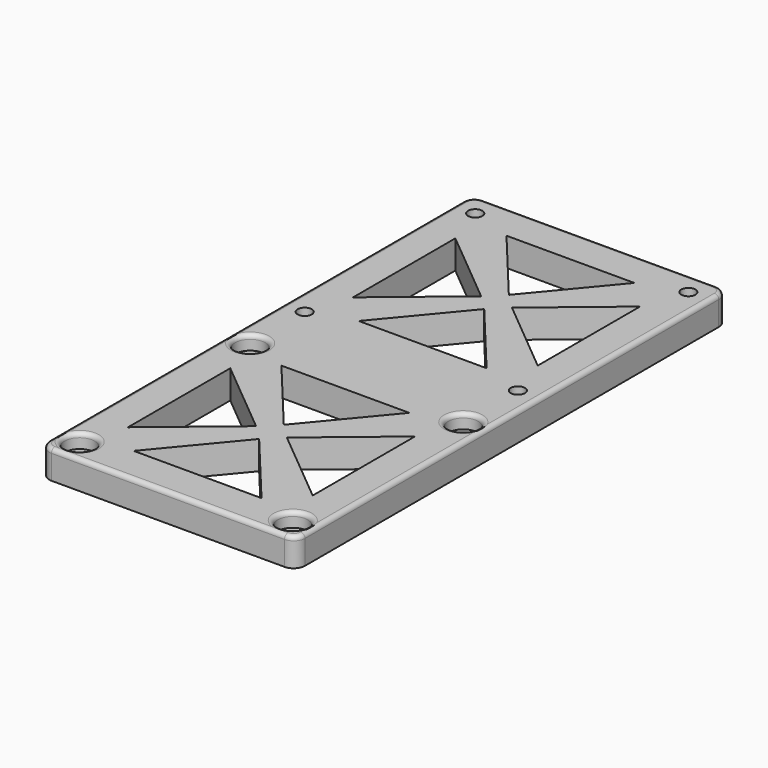
from build123d import *

# Parameters (mm, degrees)
F0_W         = 90
F0_H         = 190
F0_R         = 2.5
F1_DEPTH     = 10
F2_R         = 5.25
F3_DEPTH     = 5
F4_T1_DEPTH  = 197.5
F4_T3_DEPTH  = 97.5
F5_T1_DEPTH  = 19.9999999999
F5_T4_ANGLE  = 90
F5_T6_ANGLE  = 90
F5_T8_ANGLE  = 90
F5_T10_ANGLE = 90
F7_DEPTH     = 10


# Not quite as in the source:
# - a fillet or chamfer that OpenCascade refuses, or shapes differently, is made with other operations: its cross-section is extruded or revolved along the edge and cut away or added


with BuildPart() as f1:
    # F0 (on Top) → F1 (new body)
    with BuildSketch(Plane.XY):
        Rectangle(F0_W, F0_H)
        with Locations((-37.5, -87)):
            Circle(F0_R, mode=Mode.SUBTRACT)
        with Locations((-37.5, -12)):
            Circle(F0_R, mode=Mode.SUBTRACT)
        with Locations((37.5, -87)):
            Circle(F0_R, mode=Mode.SUBTRACT)
        with Locations((37.5, -12)):
            Circle(F0_R, mode=Mode.SUBTRACT)
        with Locations((-37.5, 12)):
            Circle(F0_R, mode=Mode.SUBTRACT)
        with Locations((-37.5, 87)):
            Circle(F0_R, mode=Mode.SUBTRACT)
        with Locations((37.5, 12)):
            Circle(F0_R, mode=Mode.SUBTRACT)
        with Locations((37.5, 87)):
            Circle(F0_R, mode=Mode.SUBTRACT)
    extrude(amount=F1_DEPTH)

    # F2 (on face) → F3 (cut)
    with BuildSketch(Plane.XY.offset(10)):
        with Locations((-37.5, -12)):
            Circle(F2_R)
        with Locations((-37.5, -87)):
            Circle(F2_R)
        with Locations((37.5, -12)):
            Circle(F2_R)
        with Locations((37.5, -87)):
            Circle(F2_R)
    extrude(amount=-F3_DEPTH, mode=Mode.SUBTRACT)

    # F4: fillet of radius 1.5 on 8 edges, made by hand

    # F4_s2 → F4_t1 (cut)
    with BuildSketch(Plane.XZ.offset(-98.75)):
        with BuildLine():
            ThreePointArc((-45, 8.5), (-44.5606601718, 9.5606601718), (-43.5, 10))
            Line((-43.5, 10), (-45, 10))
            Line((-45, 10), (-45, 8.5))
        make_face()
        with BuildLine():
            ThreePointArc((45, 8.5), (44.5606601718, 9.5606601718), (43.5, 10))
            Line((43.5, 10), (45, 10))
            Line((45, 10), (45, 8.5))
        make_face()
    extrude(amount=F4_T1_DEPTH, mode=Mode.SUBTRACT)

    # F4_s4 → F4_t3 (cut)
    with BuildSketch(Plane.YZ.offset(-48.75)):
        with BuildLine():
            ThreePointArc((93.5, 10), (94.5606601718, 9.5606601718), (95, 8.5))
            Line((95, 8.5), (95, 10))
            Line((95, 10), (93.5, 10))
        make_face()
        with BuildLine():
            ThreePointArc((-95, 8.5), (-94.5606601718, 9.5606601718), (-93.5, 10))
            Line((-93.5, 10), (-95, 10))
            Line((-95, 10), (-95, 8.5))
        make_face()
    extrude(amount=F4_T3_DEPTH, mode=Mode.SUBTRACT)

    # F4_s5 → F4_t6 (revolve, cut)
    with BuildSketch(Plane.XZ.offset(87)):
        with BuildLine():
            ThreePointArc((-30.75, 10), (-31.8106601718, 9.5606601718), (-32.25, 8.5))
            Line((-32.25, 8.5), (-32.25, 10))
            Line((-32.25, 10), (-30.75, 10))
        make_face()
    revolve(axis=Axis((-37.5, -87, 10), (0, 0, 1)), mode=Mode.SUBTRACT)

    # F4_s7 → F4_t8 (revolve, cut)
    with BuildSketch(Plane.XZ.offset(12)):
        with BuildLine():
            ThreePointArc((-30.75, 10), (-31.8106601718, 9.5606601718), (-32.25, 8.5))
            Line((-32.25, 8.5), (-32.25, 10))
            Line((-32.25, 10), (-30.75, 10))
        make_face()
    revolve(axis=Axis((-37.5, -12, 10), (0, 0, 1)), mode=Mode.SUBTRACT)

    # F4_s9 → F4_t10 (revolve, cut)
    with BuildSketch(Plane.XZ.offset(12)):
        with BuildLine():
            ThreePointArc((44.25, 10), (43.1893398282, 9.5606601718), (42.75, 8.5))
            Line((42.75, 8.5), (42.75, 10))
            Line((42.75, 10), (44.25, 10))
        make_face()
    revolve(axis=Axis((37.5, -12, 10), (0, 0, 1)), mode=Mode.SUBTRACT)

    # F4_s11 → F4_t12 (revolve, cut)
    with BuildSketch(Plane.XZ.offset(87)):
        with BuildLine():
            ThreePointArc((44.25, 10), (43.1893398282, 9.5606601718), (42.75, 8.5))
            Line((42.75, 8.5), (42.75, 10))
            Line((42.75, 10), (44.25, 10))
        make_face()
    revolve(axis=Axis((37.5, -87, 10), (0, 0, 1)), mode=Mode.SUBTRACT)

    # F5: fillet of radius 4 on 4 edges, made by hand

    # F5_s2 → F5_t1 (cut)
    with BuildSketch(Plane.XY.offset(-10)):
        with BuildLine():
            ThreePointArc((-41, -95), (-43.8284271247, -93.8284271247), (-45, -91))
            Line((-45, -91), (-45, -95))
            Line((-45, -95), (-41, -95))
        make_face()
        with BuildLine():
            ThreePointArc((41, -95), (43.8284271247, -93.8284271247), (45, -91))
            Line((45, -91), (45, -95))
            Line((45, -95), (41, -95))
        make_face()
        with BuildLine():
            ThreePointArc((45, 91), (43.8284271247, 93.8284271247), (41, 95))
            Line((41, 95), (45, 95))
            Line((45, 95), (45, 91))
        make_face()
        with BuildLine():
            ThreePointArc((-45, 91), (-43.8284271247, 93.8284271247), (-41, 95))
            Line((-41, 95), (-45, 95))
            Line((-45, 95), (-45, 91))
        make_face()
    extrude(amount=F5_T1_DEPTH, mode=Mode.SUBTRACT)

    # F5_s3 → F5_t4 (revolve, cut)
    with BuildSketch(Plane.YZ.offset(-41)):
        with BuildLine():
            ThreePointArc((93.5000000001, 10), (94.5606601718, 9.5606601718), (95, 8.5000000001))
            Line((95, 8.5000000001), (95, 10))
            Line((95, 10), (93.5000000001, 10))
        make_face()
    revolve(axis=Axis((-41, 91, 10), (0, 0, 1)), revolution_arc=F5_T4_ANGLE, mode=Mode.SUBTRACT)

    # F5_s5 → F5_t6 (revolve, cut)
    with BuildSketch(Plane.XZ.offset(-91)):
        with BuildLine():
            ThreePointArc((43.5000000001, 10), (44.5606601718, 9.5606601718), (45, 8.5000000001))
            Line((45, 8.5000000001), (45, 10))
            Line((45, 10), (43.5000000001, 10))
        make_face()
    revolve(axis=Axis((41, 91, 10), (0, 0, 1)), revolution_arc=F5_T6_ANGLE, mode=Mode.SUBTRACT)

    # F5_s7 → F5_t8 (revolve, cut)
    with BuildSketch(Plane.YZ.offset(41)):
        with BuildLine():
            ThreePointArc((-93.5000000001, 10), (-94.5606601718, 9.5606601718), (-95, 8.5000000001))
            Line((-95, 8.5000000001), (-95, 10))
            Line((-95, 10), (-93.5000000001, 10))
        make_face()
    revolve(axis=Axis((41, -91, 10), (0, 0, 1)), revolution_arc=F5_T8_ANGLE, mode=Mode.SUBTRACT)

    # F5_s9 → F5_t10 (revolve, cut)
    with BuildSketch(Plane.XZ.offset(91)):
        with BuildLine():
            ThreePointArc((-43.5000000001, 10), (-44.5606601718, 9.5606601718), (-45, 8.5000000001))
            Line((-45, 8.5000000001), (-45, 10))
            Line((-45, 10), (-43.5000000001, 10))
        make_face()
    revolve(axis=Axis((-41, -91, 10), (0, 0, 1)), revolution_arc=F5_T10_ANGLE, mode=Mode.SUBTRACT)

    # F6 (on face) → F7 (cut, through all)
    with BuildSketch(Plane.XY.offset(10)):
        Polygon((0, -44.0834977552), (22.5, -17), (-22.5, -17), align=None)
        Polygon((-5.4165022448, -49.5), (-32.5, -27), (-32.5, -72), align=None)
        Polygon((0, -54.9165022448), (-22.5, -82), (22.5, -82), align=None)
        Polygon((5.4165022448, -49.5), (32.5, -72), (32.5, -27), align=None)
        Polygon((-22.5, 17), (22.5, 17), (0, 44.0834977552), align=None)
        Polygon((32.5, 27), (32.5, 72), (5.4165022448, 49.5), align=None)
        Polygon((22.5, 82), (-22.5, 82), (0, 54.9165022448), align=None)
        Polygon((-32.5, 72), (-32.5, 27), (-5.4165022448, 49.5), align=None)
    extrude(amount=-F7_DEPTH, mode=Mode.SUBTRACT)


solid = f1.part
